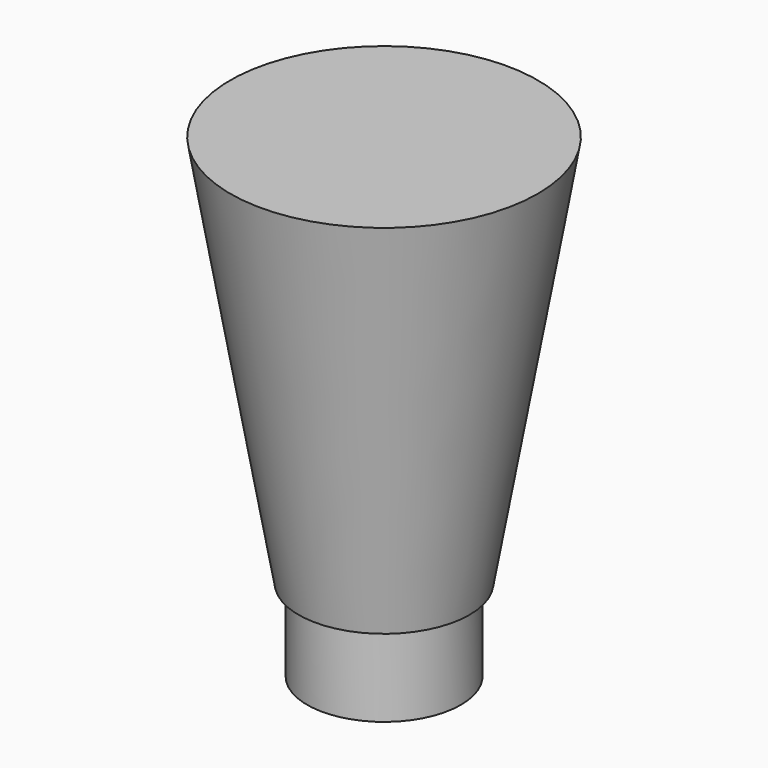
from build123d import *

# Parameters (mm, degrees)
F0_R     = 45
F1_DEPTH = 115
F2_R     = 22.5
F3_DEPTH = 24
F4_SIZE2 = 114.99999
F4_SIZE  = 19.99999


# Not quite as in the source:
# - a fillet or chamfer is up to 0.001 mm smaller than in the source, because OpenCascade refuses the exact size


with BuildPart() as f1:
    # F0 (on Top) → F1 (new body)
    with BuildSketch(Plane.XY):
        Circle(F0_R)
    extrude(amount=F1_DEPTH)

    # F2 (on face) → F3 (join)
    with BuildSketch(Plane(origin=(0, 0, 0), x_dir=(1, 0, 0), z_dir=(0, 0, -1))):
        Circle(F2_R)
    extrude(amount=F3_DEPTH)

    # F4 (size 20 and 115 in the source; OpenCascade refuses exactly that, so slightly less here)
    f4_edges = [f1.edges().sort_by_distance(p)[0] for p in [
        (-45, 0, 0),
    ]]
    f4_side = f1.faces().sort_by_distance((-43.727208, 0, 0))[0]
    chamfer(f4_edges, length=F4_SIZE, length2=F4_SIZE2, reference=f4_side)


solid = f1.part
